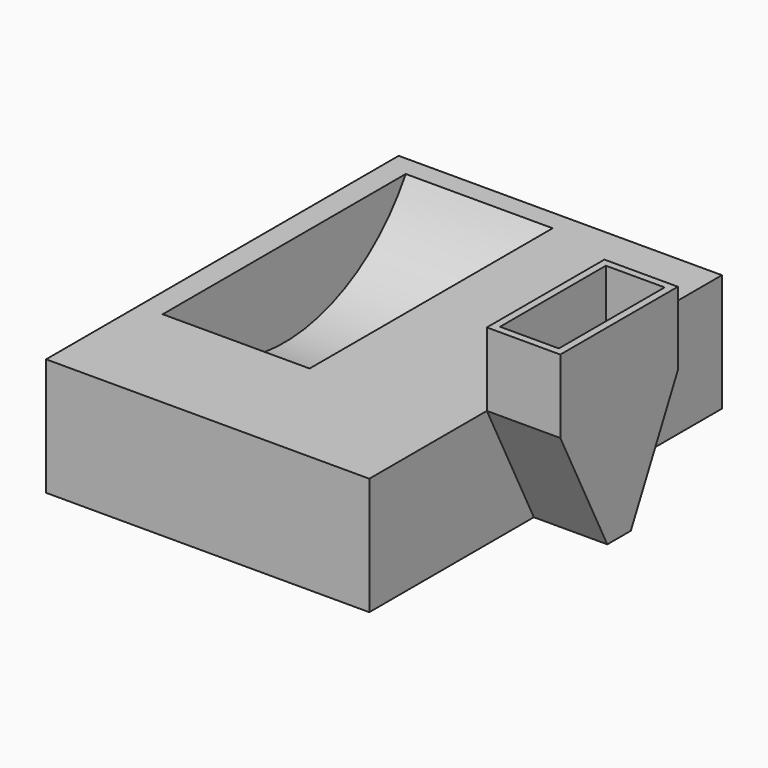
from build123d import *

# Parameters (mm, degrees)
F0_W         = 110
F0_H         = 150
F1_DEPTH     = 40
F3_R         = 60
F4_DEPTH     = 50
F6_DEPTH     = 25
F7_W         = 25
F7_H         = 50
F8_DEPTH     = 25
F9_T         = 2.5
F9_T3_DEPTH  = 49.72135955
F9_T5_DEPTH  = 55
F9_T7_DEPTH  = 49.72135955
F9_T10_ANGLE = 118.9875137878
F9_T12_ANGLE = 118.9875137878


# Not quite as in the source:
# - a shell that OpenCascade refuses in one call is made with other operations: the cavity is built on its own and cut out


with BuildPart() as f1:
    # F0 (on Top) → F1 (new body)
    with BuildSketch(Plane.XY):
        Rectangle(F0_W, F0_H)
    extrude(amount=F1_DEPTH)

    # F3 (on offset) → F4 (cut)
    with BuildSketch(Plane.YZ.offset(-47)):
        with Locations((16.3003693058, 70.4579347266)):
            Circle(F3_R)
    extrude(amount=F4_DEPTH, mode=Mode.SUBTRACT)

    # F5 (on face) → F6 (join)
    with BuildSketch(Plane.YZ.offset(55)):
        Polygon((-5, 0), (5, 0), (25, 40), (-25, 40), align=None)
    extrude(amount=F6_DEPTH)

    # F7 (on face) → F8 (join)
    with BuildSketch(Plane.XY.offset(40)):
        with Locations((67.5, 0)):
            Rectangle(F7_W, F7_H)
    extrude(amount=F8_DEPTH)

    # F9: shell of thickness 2.5, made by hand


with BuildPart() as f9_core1:
    # F9_t2: copy of F1
    add(f1.part)

    # the walls: a layer under each face that stays
    f9_faces = [f9_core1.faces().sort_by_distance(p)[0] for p in [
        (0, -75, 20),
        (-55, 0, 20),
        (55, -40, 20),
        (12.5, 0, 0),
        (-36.6666666667, -50, 40),
        (0, 75, 20),
        (67.5, -15, 20),
        (80, 0, 32.5),
        (67.5, 15, 20),
        (55, 40, 20),
        (55, 0, 52.5),
        (3, 16.3003693058, 25.2289673633),
        (-22, 16.3003693058, 10.4579347266),
        (-47, 16.3003693058, 25.2289673633),
        (67.5, -25, 52.5),
        (67.5, 25, 52.5),
    ]]
    thicken(f9_faces, amount=-F9_T, mode=Mode.SUBTRACT)

    # F9_s4 → F9_t3 (cut)
    with BuildSketch(Plane(origin=(0, -22.1180339887, 44.2360679775), x_dir=(1, 0, 0), z_dir=(0, 0.4472135955, -0.894427191))):
        Polygon((55.025, 4.497135955), (52.5, 4.472135955), (52.5, 1.972135955), (55, 1.972135955), align=None)
    extrude(amount=F9_T3_DEPTH, mode=Mode.SUBTRACT)

    # F9_s6 → F9_t5 (cut)
    with BuildSketch(Plane.XZ.offset(-27.5)):
        Polygon((54.975, 40.025), (55, 37.5), (57.5, 37.5), (57.5, 40), align=None)
    extrude(amount=F9_T5_DEPTH, mode=Mode.SUBTRACT)

    # F9_s8 → F9_t7 (cut)
    with BuildSketch(Plane(origin=(0, -0.1180339887, -0.2360679775), x_dir=(1, 0, 0), z_dir=(0, 0.4472135955, 0.894427191))):
        Polygon((55.025, 4.497135955), (55, 1.972135955), (52.5, 1.972135955), (52.5, 4.472135955), align=None)
    extrude(amount=F9_T7_DEPTH, mode=Mode.SUBTRACT)

    # F9_s9 → F9_t10 (revolve, cut)
    with BuildSketch(Plane(origin=(0, -26.6152201498, 45.172421505), x_dir=(1, 0, 0), z_dir=(0, -0.5076322454, 0.8615738525))):
        Polygon((2.975, -10.1643084047), (5.5, -10.1893084047), (5.5, -12.6893084047), (3, -12.6893084047), align=None)
    revolve(axis=Axis((3, 16.3003693058, 70.4579347266), (1, 0, 0)), revolution_arc=F9_T10_ANGLE, mode=Mode.SUBTRACT)

    # F9_s11 → F9_t12 (revolve, cut)
    with BuildSketch(Plane(origin=(0, -26.6152201498, 45.172421505), x_dir=(1, 0, 0), z_dir=(0, -0.5076322454, 0.8615738525))):
        Polygon((-46.975, -10.1643084047), (-47, -12.6893084047), (-49.5, -12.6893084047), (-49.5, -10.1893084047), align=None)
    revolve(axis=Axis((-47, 16.3003693058, 70.4579347266), (1, 0, 0)), revolution_arc=F9_T12_ANGLE, mode=Mode.SUBTRACT)


with BuildPart() as f1_1:
    add(f1.part)

    # what is left inside the walls is the cavity
    f9_cavity = [f9_core1.part.solids().sort_by_distance(p)[0] for p in [
        (12.5, -24.166667, 2.525),
    ]]
    add(f9_cavity, mode=Mode.SUBTRACT)


solid = f1_1.part
